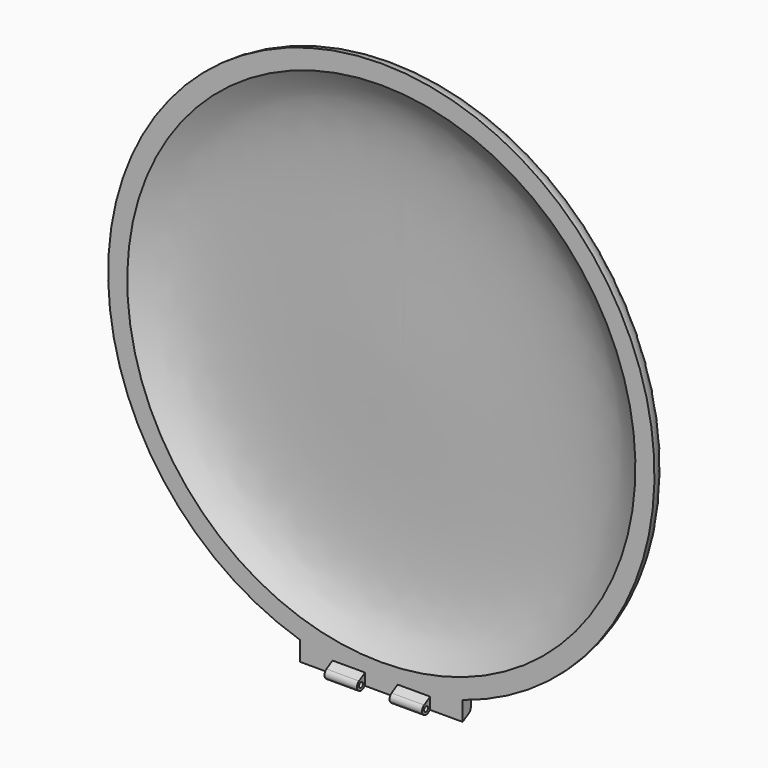
from build123d import *

# Parameters (mm, degrees)
F3_DEPTH  = 1.27
F5_DEPTH  = 20.32
F6_R      = 0.3175
F7_DEPTH  = 44.2986001
F8_R      = 0.63499
F10_W     = 4.064
F10_H     = 4.1974456223
F10_W_2   = 4.0730612593
F10_H_2   = 4.2563648137
F10_W_3   = 4.0549387407
F10_H_3   = 4.7988080594
F11_DEPTH = 1.27
F12_R     = 0.508


# Not quite as in the source:
# - a fillet or chamfer is up to 0.001 mm smaller than in the source, because OpenCascade refuses the exact size
# - the dataset's text gives a spline's control points without its knots; the knots are read off the source's solid


with BuildPart() as f1:
    # F0 (on Right) → F1 (revolve)
    with BuildSketch(Plane.YZ):
        with BuildLine():
            add(Edge.make_bspline(
                [(3.175, 0), (3.175, 10.541), (4.0422536131, 25.9599614942), (0.796980629, 30.4808964435), (0, 31.75)],
                knots=[0, 0, 0, 0, 0.6812910354, 1, 1, 1, 1], degree=3))
            Line((3.175, 0), (5.5626, 0))
            add(Edge.make_bspline(
                [(5.5626, 0), (5.5626, 1.9176420969), (5.6020893532, 5.762973782), (5.6885968485, 11.3738399623), (5.7094253413, 16.6481644408), (5.5926732239, 20.6231912945), (5.3654131178, 23.4820630282), (5.1533733603, 25.1266929623), (4.9307019402, 26.3534786039), (4.7314848723, 27.2341461126), (4.5009658464, 28.0565495549), (4.1603640769, 29.0720787187), (3.6833271227, 30.1983946783), (2.8754214133, 31.7152927686), (2.3102553011, 32.5606898933), (2.0219615984, 33.0197657478)],
                knots=[0, 0, 0, 0, 0.125, 0.25, 0.375, 0.5, 0.5625, 0.625, 0.65625, 0.6875, 0.71875, 0.75, 0.8125, 0.875, 0.9999999969, 0.9999999969, 0.9999999969, 0.9999999969], degree=3))
            ThreePointArc((2.0219615984, 33.0197657478), (1.1551928541, 33.8395366065), (0, 34.1376))
            Line((0, 34.1376), (0, 31.75))
        make_face()
    revolve(axis=Axis((0, 2.7813, 0), (0, 1, 0)))

    # F2 (on face) → F3 (join)
    with BuildSketch(Plane.XZ):
        with BuildLine():
            ThreePointArc((10.16, -30.0805069771), (0, -31.75), (-10.16, -30.0805069771))
            Line((-10.16, -30.0805069771), (-10.16, -34.2715069771))
            Line((-10.16, -34.2715069771), (10.16, -34.2715069771))
            Line((10.16, -34.2715069771), (10.16, -30.0805069771))
        make_face()
    extrude(amount=-F3_DEPTH)

    # F4 (on face) → F5 (join)
    with BuildSketch(Plane.YZ.offset(10.16)):
        Polygon((-0.8615136853, -35.5021369771), (1.27, -34.2715069771), (0.635, -33.1716547143), (-1.4965136853, -34.4022847143), align=None)
    extrude(amount=-F5_DEPTH)

    # F6 (on face) → F7 (cut, through all)
    with BuildSketch(Plane.YZ.offset(10.16)):
        with Locations((-0.635, -34.638124398)):
            Circle(F6_R)
        with BuildLine():
            Line((-0.8615136853, -35.5021369771), (-0.3175, -35.1880505294))
            ThreePointArc((-0.3175, -35.1880505294), (-0.7967279245, -35.2471937657), (-1.1790136853, -34.9522108457))
            Line((-1.1790136853, -34.9522108457), (-0.8615136853, -35.5021369771))
        make_face()
    extrude(amount=-F7_DEPTH, mode=Mode.SUBTRACT)

    # F8 (radius 0.635 in the source; OpenCascade refuses exactly that, so slightly less here)
    f8_edges = [f1.edges().sort_by_distance(p)[0] for p in [
        (0, -1.496514, -34.402285),
    ]]
    fillet(f8_edges, radius=F8_R)

    # F10 (on offset) → F11 (cut)
    with BuildSketch(Plane.XZ.offset(1.27)):
        with Locations((-8.128, -33.9503228112)):
            Rectangle(F10_W, F10_H)
        with Locations((0.0045306296, -33.9797824069)):
            Rectangle(F10_W_2, F10_H_2)
        with Locations((8.1325306296, -34.2510040297)):
            Rectangle(F10_W_3, F10_H_3)
    extrude(amount=-F11_DEPTH, mode=Mode.SUBTRACT)

    # F12
    f12_edges = [f1.edges().sort_by_distance(p)[0] for p in [
        (0, 1.27, -34.271507),
    ]]
    fillet(f12_edges, radius=F12_R)


solid = f1.part
